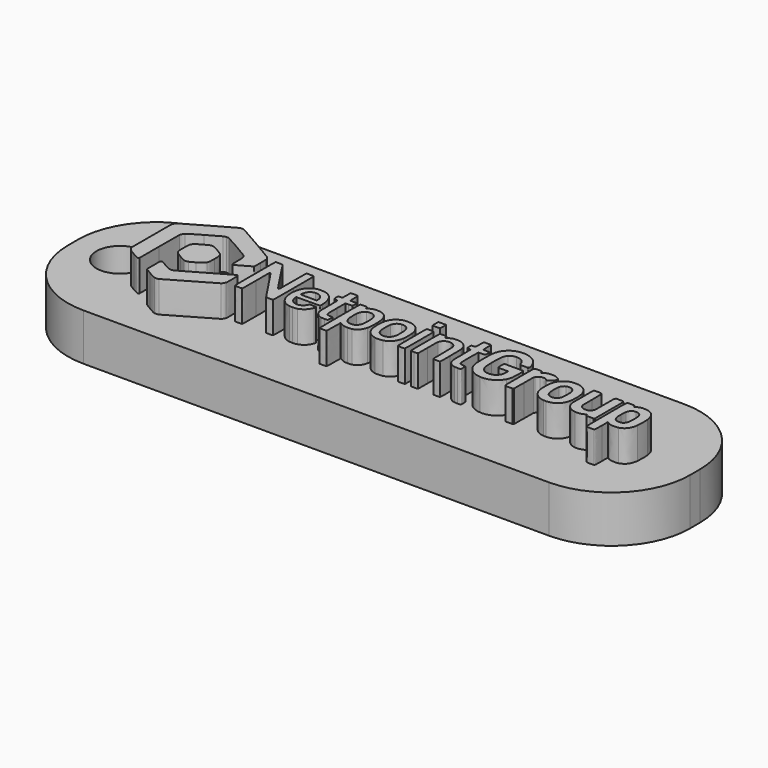
from build123d import *

# Parameters (mm, degrees)
F1_DEPTH = 2
F2_W     = 39.7300348751
F2_H     = 10.813386
F3_DEPTH = 3
F4_R     = 5
F6_D     = 3


# Not quite as in the source:
# - ends of sketch curves that miss each other by under 0.0002 mm in the source are joined
# - a feature names something its author has since deleted; it is built from what else it names


with BuildPart() as f1:
    # F0 (on Top) → F1 (new body)
    with BuildSketch(Plane.XY):
        with BuildLine():
            add(Edge.make_bspline(
                [(-12.934739, -3.423148), (-13.018761, -3.404257), (-12.980204, -3.424206), (-13.418644, -3.171907)],
                knots=[0, 0, 0, 0, 1, 1, 1, 1], degree=3))
            add(Edge.make_bspline(
                [(-12.663873, -3.404841), (-12.743201, -3.434522), (-12.851544, -3.441846), (-12.934739, -3.423148)],
                knots=[0, 0, 0, 0, 1, 1, 1, 1], degree=3))
            add(Edge.make_bspline(
                [(-9.953232, -1.835661), (-10.014995, -1.890099), (-12.572616, -3.370697), (-12.663873, -3.404841)],
                knots=[0, 0, 0, 0, 1, 1, 1, 1], degree=3))
            add(Edge.make_bspline(
                [(-9.811877, -1.614655), (-9.840102, -1.705981), (-9.884035, -1.774669), (-9.953232, -1.835661)],
                knots=[0, 0, 0, 0, 1, 1, 1, 1], degree=3))
            add(Edge.make_bspline(
                [(-9.789869, -1.125945), (-9.789869, -1.509261), (-9.791668, -1.549273), (-9.811877, -1.614655)],
                knots=[0, 0, 0, 0, 1, 1, 1, 1], degree=3))
            add(Edge.make_bspline(
                [(-9.812417, -0.679786), (-9.79074, -0.707343), (-9.789869, -0.724575), (-9.789869, -1.125945)],
                knots=[0, 0, 0, 0, 1, 1, 1, 1], degree=3))
            add(Edge.make_bspline(
                [(-9.869125, -0.643621), (-9.850334, -0.647748), (-9.824817, -0.66402), (-9.812417, -0.679786)],
                knots=[0, 0, 0, 0, 1, 1, 1, 1], degree=3))
            add(Edge.make_bspline(
                [(-11.375308, -1.483263), (-9.765318, -0.553623), (-9.910471, -0.63454), (-9.869125, -0.643621)],
                knots=[0, 0, 0, 0, 1, 1, 1, 1], degree=3))
            add(Edge.make_bspline(
                [(-12.691896, -2.226019), (-12.652934, -2.214563), (-12.167761, -1.940841), (-11.375308, -1.483263)],
                knots=[0, 0, 0, 0, 1, 1, 1, 1], degree=3))
            add(Edge.make_bspline(
                [(-12.983912, -2.221019), (-12.905986, -2.248681), (-12.776437, -2.250898), (-12.691896, -2.226019)],
                knots=[0, 0, 0, 0, 1, 1, 1, 1], degree=3))
            add(Edge.make_bspline(
                [(-13.358996, -2.018025), (-13.186933, -2.117519), (-13.018145, -2.208866), (-12.983912, -2.221019)],
                knots=[0, 0, 0, 0, 1, 1, 1, 1], degree=3))
            add(Edge.make_bspline(
                [(-13.768617, -1.851494), (-13.721476, -1.815301), (-13.68144, -1.831571), (-13.358996, -2.018025)],
                knots=[0, 0, 0, 0, 1, 1, 1, 1], degree=3))
            add(Edge.make_bspline(
                [(-13.812466, -2.408405), (-13.812466, -1.902548), (-13.81101, -1.88404), (-13.768617, -1.851494)],
                knots=[0, 0, 0, 0, 1, 1, 1, 1], degree=3))
            add(Edge.make_bspline(
                [(-13.796813, -2.932975), (-13.809518, -2.908422), (-13.812466, -2.809669), (-13.812466, -2.408405)],
                knots=[0, 0, 0, 0, 1, 1, 1, 1], degree=3))
            add(Edge.make_bspline(
                [(-13.418644, -3.171907), (-13.685045, -3.01856), (-13.785311, -2.955211), (-13.796813, -2.932975)],
                knots=[0, 0, 0, 0, 1, 1, 1, 1], degree=3))
        make_face()
    extrude(amount=F1_DEPTH)



with BuildPart() as f1b:
    # F0 (on Top) → F1, piece 2 (new body)
    with BuildSketch(Plane.XY):
        with BuildLine():
            add(Edge.make_bspline(
                [(-3.094246, -2.529348), (-3.109835, -2.507097), (-3.11169, -2.335221), (-3.11169, -0.912718)],
                knots=[0, 0, 0, 0, 1, 1, 1, 1], degree=3))
            add(Edge.make_bspline(
                [(-2.870782, -2.554235), (-3.070978, -2.554235), (-3.077297, -2.553441), (-3.094246, -2.529348)],
                knots=[0, 0, 0, 0, 1, 1, 1, 1], degree=3))
            add(Edge.make_bspline(
                [(-2.647318, -2.529338), (-2.664267, -2.553547), (-2.670588, -2.554235), (-2.870782, -2.554235)],
                knots=[0, 0, 0, 0, 1, 1, 1, 1], degree=3))
            add(Edge.make_bspline(
                [(-2.629874, -1.993739), (-2.629874, -2.437824), (-2.632149, -2.507682), (-2.647318, -2.529338)],
                knots=[0, 0, 0, 0, 1, 1, 1, 1], degree=3))
            add(Edge.make_bspline(
                [(-2.616427, -1.469597), (-2.626492, -1.479651), (-2.629874, -1.611472), (-2.629874, -1.993739)],
                knots=[0, 0, 0, 0, 1, 1, 1, 1], degree=3))
            add(Edge.make_bspline(
                [(-2.519436, -1.488038), (-2.563105, -1.453941), (-2.59475, -1.447927), (-2.616427, -1.469597)],
                knots=[0, 0, 0, 0, 1, 1, 1, 1], degree=3))
            add(Edge.make_bspline(
                [(-2.293723, -1.603719), (-2.382754, -1.576049), (-2.452487, -1.540309), (-2.519436, -1.488038)],
                knots=[0, 0, 0, 0, 1, 1, 1, 1], degree=3))
            add(Edge.make_bspline(
                [(-2.030406, -1.629622), (-2.187038, -1.629834), (-2.220303, -1.626526), (-2.293723, -1.603719)],
                knots=[0, 0, 0, 0, 1, 1, 1, 1], degree=3))
            add(Edge.make_bspline(
                [(-1.778293, -1.609276), (-1.834176, -1.624727), (-1.892849, -1.629463), (-2.030406, -1.629622)],
                knots=[0, 0, 0, 0, 1, 1, 1, 1], degree=3))
            add(Edge.make_bspline(
                [(-1.247316, -1.022649), (-1.323597, -1.33902), (-1.498066, -1.531777), (-1.778293, -1.609276)],
                knots=[0, 0, 0, 0, 1, 1, 1, 1], degree=3))
            add(Edge.make_bspline(
                [(-1.198527, -0.360448), (-1.192326, -0.683075), (-1.204155, -0.84364), (-1.247316, -1.022649)],
                knots=[0, 0, 0, 0, 1, 1, 1, 1], degree=3))
            add(Edge.make_bspline(
                [(-1.26407, 0.207777), (-1.217128, 0.049678), (-1.204268, -0.061812), (-1.198527, -0.360448)],
                knots=[0, 0, 0, 0, 1, 1, 1, 1], degree=3))
            add(Edge.make_bspline(
                [(-1.621423, 0.665032), (-1.461517, 0.588518), (-1.325404, 0.41435), (-1.26407, 0.207777)],
                knots=[0, 0, 0, 0, 1, 1, 1, 1], degree=3))
            add(Edge.make_bspline(
                [(-1.987661, 0.748273), (-1.821812, 0.742108), (-1.746889, 0.725069), (-1.621423, 0.665032)],
                knots=[0, 0, 0, 0, 1, 1, 1, 1], degree=3))
            add(Edge.make_bspline(
                [(-2.505454, 0.613399), (-2.363918, 0.720529), (-2.223672, 0.75706), (-1.987661, 0.748273)],
                knots=[0, 0, 0, 0, 1, 1, 1, 1], degree=3))
            add(Edge.make_bspline(
                [(-2.607019, 0.568018), (-2.582645, 0.559498), (-2.568071, 0.565901), (-2.505454, 0.613399)],
                knots=[0, 0, 0, 0, 1, 1, 1, 1], degree=3))
            add(Edge.make_bspline(
                [(-2.639002, 0.633698), (-2.635959, 0.585607), (-2.631575, 0.576603), (-2.607019, 0.568018)],
                knots=[0, 0, 0, 0, 1, 1, 1, 1], degree=3))
            add(Edge.make_bspline(
                [(-2.877485, 0.72881), (-2.648098, 0.72881), (-2.644941, 0.727487), (-2.639002, 0.633698)],
                knots=[0, 0, 0, 0, 1, 1, 1, 1], degree=3))
            add(Edge.make_bspline(
                [(-3.094246, 0.703913), (-3.077331, 0.728069), (-3.070753, 0.72881), (-2.877485, 0.72881)],
                knots=[0, 0, 0, 0, 1, 1, 1, 1], degree=3))
            add(Edge.make_bspline(
                [(-3.11169, -0.912718), (-3.11169, 0.509783), (-3.109837, 0.681656), (-3.094246, 0.703913)],
                knots=[0, 0, 0, 0, 1, 1, 1, 1], degree=3))
        make_face()
        with BuildLine():
            add(Edge.make_bspline(
                [(-1.991503, -1.191898), (-1.747455, -1.119423), (-1.652635, -0.872662), (-1.669226, -0.353201)],
                knots=[0, 0, 0, 0, 1, 1, 1, 1], degree=3))
            add(Edge.make_bspline(
                [(-2.323383, -1.186519), (-2.235741, -1.2143), (-2.07574, -1.216875), (-1.991503, -1.191898)],
                knots=[0, 0, 0, 0, 1, 1, 1, 1], degree=3))
            add(Edge.make_bspline(
                [(-2.602575, -0.82304), (-2.560305, -1.010558), (-2.457898, -1.143881), (-2.323383, -1.186519)],
                knots=[0, 0, 0, 0, 1, 1, 1, 1], degree=3))
            add(Edge.make_bspline(
                [(-2.618942, -0.170408), (-2.637084, -0.315021), (-2.62707, -0.714373), (-2.602575, -0.82304)],
                knots=[0, 0, 0, 0, 1, 1, 1, 1], degree=3))
            add(Edge.make_bspline(
                [(-2.357878, 0.291896), (-2.505464, 0.226613), (-2.58732, 0.081658), (-2.618942, -0.170408)],
                knots=[0, 0, 0, 0, 1, 1, 1, 1], degree=3))
            add(Edge.make_bspline(
                [(-1.939523, 0.292425), (-2.052117, 0.34223), (-2.24459, 0.341968), (-2.357878, 0.291896)],
                knots=[0, 0, 0, 0, 1, 1, 1, 1], degree=3))
            add(Edge.make_bspline(
                [(-1.747097, 0.092964), (-1.786426, 0.179112), (-1.863151, 0.258643), (-1.939523, 0.292425)],
                knots=[0, 0, 0, 0, 1, 1, 1, 1], degree=3))
            add(Edge.make_bspline(
                [(-1.669226, -0.353201), (-1.67619, -0.135176), (-1.696766, -0.017286), (-1.747097, 0.092964)],
                knots=[0, 0, 0, 0, 1, 1, 1, 1], degree=3))
        make_face(mode=Mode.SUBTRACT)
    extrude(amount=F1_DEPTH)


with BuildPart() as f1c:
    # F0 (on Top) → F1, piece 3 (new body)
    with BuildSketch(Plane.XY):
        with BuildLine():
            add(Edge.make_bspline(
                [(13.969443, -2.530221), (13.956637, -2.524004), (13.937716, -2.504663), (13.927424, -2.487232)],
                knots=[0, 0, 0, 0, 1, 1, 1, 1], degree=3))
            add(Edge.make_bspline(
                [(14.418843, -2.529645), (14.382354, -2.54626), (14.003518, -2.546737), (13.969443, -2.530221)],
                knots=[0, 0, 0, 0, 1, 1, 1, 1], degree=3))
            add(Edge.make_bspline(
                [(14.48016, -1.966548), (14.48016, -2.495815), (14.479366, -2.502014), (14.418843, -2.529645)],
                knots=[0, 0, 0, 0, 1, 1, 1, 1], degree=3))
            Line((14.48016, -1.966548), (14.48016, -1.478593))
            Line((14.48016, -1.478593), (14.533383, -1.516449))
            add(Edge.make_bspline(
                [(15.012396, -1.649048), (14.793157, -1.649048), (14.673065, -1.615803), (14.533383, -1.516449)],
                knots=[0, 0, 0, 0, 1, 1, 1, 1], degree=3))
            add(Edge.make_bspline(
                [(15.258905, -1.625447), (15.188222, -1.644074), (15.136094, -1.649048), (15.012396, -1.649048)],
                knots=[0, 0, 0, 0, 1, 1, 1, 1], degree=3))
            add(Edge.make_bspline(
                [(15.855107, -0.856687), (15.786633, -1.29838), (15.603337, -1.534729), (15.258905, -1.625447)],
                knots=[0, 0, 0, 0, 1, 1, 1, 1], degree=3))
            add(Edge.make_bspline(
                [(15.860557, -0.049927), (15.882306, -0.204735), (15.878946, -0.703062), (15.855107, -0.856687)],
                knots=[0, 0, 0, 0, 1, 1, 1, 1], degree=3))
            add(Edge.make_bspline(
                [(15.292534, 0.740399), (15.625806, 0.634193), (15.798171, 0.394372), (15.860557, -0.049927)],
                knots=[0, 0, 0, 0, 1, 1, 1, 1], degree=3))
            add(Edge.make_bspline(
                [(14.785685, 0.753311), (14.910825, 0.784955), (15.173715, 0.778261), (15.292534, 0.740399)],
                knots=[0, 0, 0, 0, 1, 1, 1, 1], degree=3))
            add(Edge.make_bspline(
                [(14.520824, 0.632917), (14.591428, 0.686829), (14.677499, 0.725953), (14.785685, 0.753311)],
                knots=[0, 0, 0, 0, 1, 1, 1, 1], degree=3))
            Line((14.520824, 0.632917), (14.468968, 0.593322))
            Line((14.468968, 0.593322), (14.468968, 0.639519))
            add(Edge.make_bspline(
                [(14.436213, 0.718465), (14.461824, 0.692853), (14.468968, 0.675637), (14.468968, 0.639519)],
                knots=[0, 0, 0, 0, 1, 1, 1, 1], degree=3))
            Line((14.436213, 0.718465), (14.40346, 0.75122))
            Line((14.40346, 0.75122), (14.201437, 0.75122))
            add(Edge.make_bspline(
                [(13.971411, 0.738468), (13.989032, 0.746511), (14.074228, 0.75122), (14.201437, 0.75122)],
                knots=[0, 0, 0, 0, 1, 1, 1, 1], degree=3))
            add(Edge.make_bspline(
                [(13.908718, -0.901478), (13.908718, 0.796102), (13.905358, 0.708374), (13.971411, 0.738468)],
                knots=[0, 0, 0, 0, 1, 1, 1, 1], degree=3))
            add(Edge.make_bspline(
                [(13.927424, -2.487232), (13.910173, -2.458046), (13.908718, -2.333144), (13.908718, -0.901478)],
                knots=[0, 0, 0, 0, 1, 1, 1, 1], degree=3))
        make_face()
        with BuildLine():
            add(Edge.make_bspline(
                [(15.075031, -1.101257), (15.176363, -1.055513), (15.239564, -0.966142), (15.283649, -0.806271)],
                knots=[0, 0, 0, 0, 1, 1, 1, 1], degree=3))
            add(Edge.make_bspline(
                [(14.911492, -1.127763), (14.995505, -1.125382), (15.036409, -1.118661), (15.075031, -1.101257)],
                knots=[0, 0, 0, 0, 1, 1, 1, 1], degree=3))
            add(Edge.make_bspline(
                [(14.641961, -1.049901), (14.714782, -1.113999), (14.776184, -1.131737), (14.911492, -1.127763)],
                knots=[0, 0, 0, 0, 1, 1, 1, 1], degree=3))
            add(Edge.make_bspline(
                [(14.511746, -0.822111), (14.541808, -0.93136), (14.57677, -0.992516), (14.641961, -1.049901)],
                knots=[0, 0, 0, 0, 1, 1, 1, 1], degree=3))
            add(Edge.make_bspline(
                [(14.486637, -0.442109), (14.487166, -0.705406), (14.489706, -0.741969), (14.511746, -0.822111)],
                knots=[0, 0, 0, 0, 1, 1, 1, 1], degree=3))
            add(Edge.make_bspline(
                [(14.50566, -0.07342), (14.489177, -0.137981), (14.486028, -0.198967), (14.486637, -0.442109)],
                knots=[0, 0, 0, 0, 1, 1, 1, 1], degree=3))
            add(Edge.make_bspline(
                [(14.874177, 0.255862), (14.667548, 0.245226), (14.563184, 0.151982), (14.50566, -0.07342)],
                knots=[0, 0, 0, 0, 1, 1, 1, 1], degree=3))
            add(Edge.make_bspline(
                [(15.157713, 0.166886), (15.078131, 0.239617), (15.004935, 0.262588), (14.874177, 0.255862)],
                knots=[0, 0, 0, 0, 1, 1, 1, 1], degree=3))
            add(Edge.make_bspline(
                [(15.284178, -0.069083), (15.250261, 0.053554), (15.220065, 0.1099), (15.157713, 0.166886)],
                knots=[0, 0, 0, 0, 1, 1, 1, 1], degree=3))
            add(Edge.make_bspline(
                [(15.283649, -0.806271), (15.312886, -0.700241), (15.313304, -0.174189), (15.284178, -0.069083)],
                knots=[0, 0, 0, 0, 1, 1, 1, 1], degree=3))
        make_face(mode=Mode.SUBTRACT)
    extrude(amount=F1_DEPTH)


with BuildPart() as f1d:
    # F0 (on Top) → F1, piece 4 (new body)
    with BuildSketch(Plane.XY):
        with BuildLine():
            add(Edge.make_bspline(
                [(-15.319538, -2.078617), (-15.580275, -1.928162), (-15.670973, -1.869888), (-15.723821, -1.818868)],
                knots=[0, 0, 0, 0, 1, 1, 1, 1], degree=3))
            add(Edge.make_bspline(
                [(-14.870841, -2.246633), (-14.925169, -2.30096), (-14.95105, -2.291268), (-15.319538, -2.078617)],
                knots=[0, 0, 0, 0, 1, 1, 1, 1], degree=3))
            Line((-14.870841, -2.246633), (-14.843339, -2.21913))
            Line((-14.843339, -2.21913), (-14.843339, -0.657051))
            add(Edge.make_bspline(
                [(-14.832075, 0.965382), (-14.839283, 0.926769), (-14.843339, 0.34231), (-14.843339, -0.657051)],
                knots=[0, 0, 0, 0, 1, 1, 1, 1], degree=3))
            add(Edge.make_bspline(
                [(-14.693636, 1.223883), (-14.759078, 1.160351), (-14.815271, 1.055422), (-14.832075, 0.965382)],
                knots=[0, 0, 0, 0, 1, 1, 1, 1], degree=3))
            add(Edge.make_bspline(
                [(-13.879709, 1.716952), (-14.456598, 1.383514), (-14.64971, 1.266528), (-14.693636, 1.223883)],
                knots=[0, 0, 0, 0, 1, 1, 1, 1], degree=3))
            add(Edge.make_bspline(
                [(-13.04001, 2.194448), (-13.08586, 2.172276), (-13.463724, 1.957392), (-13.879709, 1.716952)],
                knots=[0, 0, 0, 0, 1, 1, 1, 1], degree=3))
            add(Edge.make_bspline(
                [(-12.85963, 2.239422), (-12.942676, 2.235454), (-12.968655, 2.228971), (-13.04001, 2.194448)],
                knots=[0, 0, 0, 0, 1, 1, 1, 1], degree=3))
            add(Edge.make_bspline(
                [(-12.69648, 2.225029), (-12.743918, 2.238681), (-12.790032, 2.242756), (-12.85963, 2.239422)],
                knots=[0, 0, 0, 0, 1, 1, 1, 1], degree=3))
            add(Edge.make_bspline(
                [(-10.982981, 1.24161), (-11.057248, 1.306859), (-12.617411, 2.202275), (-12.69648, 2.225029)],
                knots=[0, 0, 0, 0, 1, 1, 1, 1], degree=3))
            add(Edge.make_bspline(
                [(-10.841973, 1.019116), (-10.868471, 1.104254), (-10.921021, 1.187172), (-10.982981, 1.24161)],
                knots=[0, 0, 0, 0, 1, 1, 1, 1], degree=3))
            add(Edge.make_bspline(
                [(-10.820745, 0.57038), (-10.820745, 0.912378), (-10.822889, 0.957815), (-10.841973, 1.019116)],
                knots=[0, 0, 0, 0, 1, 1, 1, 1], degree=3))
            add(Edge.make_bspline(
                [(-10.804778, 0.158974), (-10.817679, 0.183925), (-10.820745, 0.26295), (-10.820745, 0.57038)],
                knots=[0, 0, 0, 0, 1, 1, 1, 1], degree=3))
            add(Edge.make_bspline(
                [(-10.711785, 0.101324), (-10.745788, 0.101324), (-10.788733, 0.127949), (-10.804778, 0.158974)],
                knots=[0, 0, 0, 0, 1, 1, 1, 1], degree=3))
            add(Edge.make_bspline(
                [(-9.80938, 0.61967), (-9.838929, 0.590121), (-10.689892, 0.101324), (-10.711785, 0.101324)],
                knots=[0, 0, 0, 0, 1, 1, 1, 1], degree=3))
            add(Edge.make_bspline(
                [(-9.792129, 1.119346), (-9.788957, 0.666673), (-9.789907, 0.63914), (-9.80938, 0.61967)],
                knots=[0, 0, 0, 0, 1, 1, 1, 1], degree=3))
            Line((-9.792129, 1.119346), (-9.795487, 1.598416))
            Line((-9.795487, 1.598416), (-9.837583, 1.683562))
            add(Edge.make_bspline(
                [(-9.94403, 1.82731), (-9.898154, 1.785532), (-9.867592, 1.74426), (-9.837583, 1.683562)],
                knots=[0, 0, 0, 0, 1, 1, 1, 1], degree=3))
            add(Edge.make_bspline(
                [(-11.30764, 2.635199), (-10.330074, 2.071433), (-9.992448, 1.871403), (-9.94403, 1.82731)],
                knots=[0, 0, 0, 0, 1, 1, 1, 1], degree=3))
            add(Edge.make_bspline(
                [(-12.669047, 3.408545), (-12.634865, 3.395315), (-12.022232, 3.047306), (-11.30764, 2.635199)],
                knots=[0, 0, 0, 0, 1, 1, 1, 1], degree=3))
            add(Edge.make_bspline(
                [(-12.98331, 3.41119), (-12.89578, 3.441845), (-12.751932, 3.440639), (-12.669047, 3.408545)],
                knots=[0, 0, 0, 0, 1, 1, 1, 1], degree=3))
            add(Edge.make_bspline(
                [(-14.221462, 2.710333), (-13.574373, 3.083933), (-13.017205, 3.399319), (-12.98331, 3.41119)],
                knots=[0, 0, 0, 0, 1, 1, 1, 1], degree=3))
            add(Edge.make_bspline(
                [(-15.532448, 1.954191), (-15.458495, 1.996466), (-14.868551, 2.336731), (-14.221462, 2.710333)],
                knots=[0, 0, 0, 0, 1, 1, 1, 1], degree=3))
            add(Edge.make_bspline(
                [(-15.861696, 1.571439), (-15.827793, 1.73243), (-15.738217, 1.836565), (-15.532448, 1.954191)],
                knots=[0, 0, 0, 0, 1, 1, 1, 1], degree=3))
            add(Edge.make_bspline(
                [(-15.861696, -1.570461), (-15.879346, -1.486551), (-15.879331, 1.48763), (-15.861696, 1.571439)],
                knots=[0, 0, 0, 0, 1, 1, 1, 1], degree=3))
            add(Edge.make_bspline(
                [(-15.723821, -1.818868), (-15.797391, -1.747843), (-15.840859, -1.669527), (-15.861696, -1.570461)],
                knots=[0, 0, 0, 0, 1, 1, 1, 1], degree=3))
        make_face()
    extrude(amount=F1_DEPTH)


with BuildPart() as f1e:
    # F0 (on Top) → F1, piece 5 (new body)
    with BuildSketch(Plane.XY):
        with BuildLine():
            add(Edge.make_bspline(
                [(6.45178, -1.650474), (6.128772, -1.624465), (5.876884, -1.508599), (5.67293, -1.292194)],
                knots=[0, 0, 0, 0, 1, 1, 1, 1], degree=3))
            add(Edge.make_bspline(
                [(7.644658, -1.01608), (7.436155, -1.441268), (6.965051, -1.691815), (6.45178, -1.650474)],
                knots=[0, 0, 0, 0, 1, 1, 1, 1], degree=3))
            add(Edge.make_bspline(
                [(7.768353, -0.19652), (7.768353, -0.670148), (7.747924, -0.80549), (7.644658, -1.01608)],
                knots=[0, 0, 0, 0, 1, 1, 1, 1], degree=3))
            Line((7.768353, -0.19652), (7.768353, 0.139313))
            Line((7.768353, 0.139313), (7.738244, 0.17074))
            Line((7.738244, 0.17074), (7.708135, 0.202165))
            Line((7.708135, 0.202165), (7.13527, 0.202165))
            Line((7.13527, 0.202165), (6.562406, 0.202165))
            Line((6.562406, 0.202165), (6.532297, 0.17074))
            Line((6.532297, 0.17074), (6.502188, 0.139313))
            Line((6.502188, 0.139313), (6.502188, -0.057968))
            Line((6.502188, -0.057968), (6.502188, -0.255247))
            Line((6.502188, -0.255247), (6.536662, -0.284256))
            Line((6.536662, -0.284256), (6.571138, -0.313264))
            Line((6.571138, -0.313264), (6.872812, -0.313264))
            Line((6.872812, -0.313264), (7.174488, -0.313264))
            Line((7.174488, -0.313264), (7.174488, -0.445932))
            add(Edge.make_bspline(
                [(7.000891, -0.936176), (7.125751, -0.80961), (7.174488, -0.671957), (7.174488, -0.445932)],
                knots=[0, 0, 0, 0, 1, 1, 1, 1], degree=3))
            add(Edge.make_bspline(
                [(6.706107, -1.096526), (6.809656, -1.075095), (6.926636, -1.01146), (7.000891, -0.936176)],
                knots=[0, 0, 0, 0, 1, 1, 1, 1], degree=3))
            add(Edge.make_bspline(
                [(6.391589, -1.092531), (6.463321, -1.111634), (6.623334, -1.113645), (6.706107, -1.096526)],
                knots=[0, 0, 0, 0, 1, 1, 1, 1], degree=3))
            add(Edge.make_bspline(
                [(6.061641, -0.852914), (6.118508, -0.957395), (6.254252, -1.055976), (6.391589, -1.092531)],
                knots=[0, 0, 0, 0, 1, 1, 1, 1], degree=3))
            add(Edge.make_bspline(
                [(5.945178, -0.100357), (5.952973, -0.560999), (5.972923, -0.689907), (6.061641, -0.852914)],
                knots=[0, 0, 0, 0, 1, 1, 1, 1], degree=3))
            add(Edge.make_bspline(
                [(6.133157, 0.986215), (5.977622, 0.83068), (5.933716, 0.576897), (5.945178, -0.100357)],
                knots=[0, 0, 0, 0, 1, 1, 1, 1], degree=3))
            add(Edge.make_bspline(
                [(6.518974, 1.150844), (6.357482, 1.141267), (6.236639, 1.089699), (6.133157, 0.986215)],
                knots=[0, 0, 0, 0, 1, 1, 1, 1], degree=3))
            add(Edge.make_bspline(
                [(6.976112, 0.99905), (6.858225, 1.111146), (6.705361, 1.161907), (6.518974, 1.150844)],
                knots=[0, 0, 0, 0, 1, 1, 1, 1], degree=3))
            add(Edge.make_bspline(
                [(7.146938, 0.725503), (7.105698, 0.842473), (7.054418, 0.924589), (6.976112, 0.99905)],
                knots=[0, 0, 0, 0, 1, 1, 1, 1], degree=3))
            add(Edge.make_bspline(
                [(7.201003, 0.621855), (7.187888, 0.631036), (7.164296, 0.676269), (7.146938, 0.725503)],
                knots=[0, 0, 0, 0, 1, 1, 1, 1], degree=3))
            add(Edge.make_bspline(
                [(7.452219, 0.605557), (7.270898, 0.605557), (7.219513, 0.60889), (7.201003, 0.621855)],
                knots=[0, 0, 0, 0, 1, 1, 1, 1], degree=3))
            add(Edge.make_bspline(
                [(7.702787, 0.617675), (7.688708, 0.610134), (7.594076, 0.605557), (7.452219, 0.605557)],
                knots=[0, 0, 0, 0, 1, 1, 1, 1], degree=3))
            add(Edge.make_bspline(
                [(7.741684, 0.668734), (7.732733, 0.647303), (7.715228, 0.624334), (7.702787, 0.617675)],
                knots=[0, 0, 0, 0, 1, 1, 1, 1], degree=3))
            add(Edge.make_bspline(
                [(7.729265, 0.816297), (7.755638, 0.716467), (7.756643, 0.704537), (7.741684, 0.668734)],
                knots=[0, 0, 0, 0, 1, 1, 1, 1], degree=3))
            add(Edge.make_bspline(
                [(7.639998, 1.048165), (7.673313, 0.980376), (7.713482, 0.876035), (7.729265, 0.816297)],
                knots=[0, 0, 0, 0, 1, 1, 1, 1], degree=3))
            add(Edge.make_bspline(
                [(6.781854, 1.676479), (7.17654, 1.607769), (7.470908, 1.39224), (7.639998, 1.048165)],
                knots=[0, 0, 0, 0, 1, 1, 1, 1], degree=3))
            add(Edge.make_bspline(
                [(6.216439, 1.654413), (6.36732, 1.693756), (6.62485, 1.703805), (6.781854, 1.676479)],
                knots=[0, 0, 0, 0, 1, 1, 1, 1], degree=3))
            add(Edge.make_bspline(
                [(5.695195, 1.357267), (5.839101, 1.50247), (6.012221, 1.60116), (6.216439, 1.654413)],
                knots=[0, 0, 0, 0, 1, 1, 1, 1], degree=3))
            add(Edge.make_bspline(
                [(5.368531, 0.627165), (5.409832, 0.951552), (5.505901, 1.166267), (5.695195, 1.357267)],
                knots=[0, 0, 0, 0, 1, 1, 1, 1], degree=3))
            add(Edge.make_bspline(
                [(5.368658, -0.592805), (5.347978, -0.429671), (5.347912, 0.464941), (5.368531, 0.627165)],
                knots=[0, 0, 0, 0, 1, 1, 1, 1], degree=3))
            add(Edge.make_bspline(
                [(5.67293, -1.292194), (5.498333, -1.106943), (5.407308, -0.897716), (5.368658, -0.592805)],
                knots=[0, 0, 0, 0, 1, 1, 1, 1], degree=3))
        make_face()
    extrude(amount=F1_DEPTH)


with BuildPart() as f1f:
    # F0 (on Top) → F1, piece 6 (new body)
    with BuildSketch(Plane.XY):
        with BuildLine():
            add(Edge.make_bspline(
                [(10.485581, -1.646955), (10.08999, -1.601179), (9.797088, -1.361583), (9.680026, -0.988002)],
                knots=[0, 0, 0, 0, 1, 1, 1, 1], degree=3))
            add(Edge.make_bspline(
                [(10.664807, -1.650572), (10.609343, -1.653588), (10.528666, -1.651895), (10.485581, -1.646955)],
                knots=[0, 0, 0, 0, 1, 1, 1, 1], degree=3))
            add(Edge.make_bspline(
                [(11.579453, -0.880843), (11.477195, -1.349378), (11.15058, -1.624243), (10.664807, -1.650572)],
                knots=[0, 0, 0, 0, 1, 1, 1, 1], degree=3))
            add(Edge.make_bspline(
                [(11.579189, 0.009271), (11.627817, -0.213532), (11.627975, -0.658771), (11.579453, -0.880843)],
                knots=[0, 0, 0, 0, 1, 1, 1, 1], degree=3))
            add(Edge.make_bspline(
                [(10.800666, 0.762923), (11.205891, 0.697555), (11.488728, 0.423754), (11.579189, 0.009271)],
                knots=[0, 0, 0, 0, 1, 1, 1, 1], degree=3))
            add(Edge.make_bspline(
                [(10.340606, 0.74636), (10.43041, 0.771151), (10.69144, 0.780549), (10.800666, 0.762923)],
                knots=[0, 0, 0, 0, 1, 1, 1, 1], degree=3))
            add(Edge.make_bspline(
                [(9.914126, 0.498842), (10.046106, 0.631174), (10.157482, 0.695811), (10.340606, 0.74636)],
                knots=[0, 0, 0, 0, 1, 1, 1, 1], degree=3))
            add(Edge.make_bspline(
                [(9.699658, 0.169108), (9.753545, 0.312568), (9.800789, 0.385204), (9.914126, 0.498842)],
                knots=[0, 0, 0, 0, 1, 1, 1, 1], degree=3))
            add(Edge.make_bspline(
                [(9.620314, -0.374886), (9.626373, -0.095512), (9.642936, 0.018118), (9.699658, 0.169108)],
                knots=[0, 0, 0, 0, 1, 1, 1, 1], degree=3))
            add(Edge.make_bspline(
                [(9.680026, -0.988002), (9.631371, -0.832726), (9.614208, -0.656506), (9.620314, -0.374886)],
                knots=[0, 0, 0, 0, 1, 1, 1, 1], degree=3))
        make_face()
        with BuildLine():
            add(Edge.make_bspline(
                [(10.795377, -1.095479), (10.914791, -1.040382), (10.983472, -0.945603), (11.025241, -0.778264)],
                knots=[0, 0, 0, 0, 1, 1, 1, 1], degree=3))
            add(Edge.make_bspline(
                [(10.460438, -1.108107), (10.546869, -1.14226), (10.707069, -1.136219), (10.795377, -1.095479)],
                knots=[0, 0, 0, 0, 1, 1, 1, 1], degree=3))
            add(Edge.make_bspline(
                [(10.206044, -0.759), (10.2384, -0.931948), (10.32889, -1.05613), (10.460438, -1.108107)],
                knots=[0, 0, 0, 0, 1, 1, 1, 1], degree=3))
            add(Edge.make_bspline(
                [(10.212473, -0.069377), (10.175101, -0.223362), (10.171807, -0.576059), (10.206044, -0.759)],
                knots=[0, 0, 0, 0, 1, 1, 1, 1], degree=3))
            add(Edge.make_bspline(
                [(10.43348, 0.222924), (10.321849, 0.17059), (10.246538, 0.070982), (10.212473, -0.069377)],
                knots=[0, 0, 0, 0, 1, 1, 1, 1], degree=3))
            add(Edge.make_bspline(
                [(10.614418, 0.252595), (10.510571, 0.252595), (10.489338, 0.249102), (10.43348, 0.222924)],
                knots=[0, 0, 0, 0, 1, 1, 1, 1], degree=3))
            add(Edge.make_bspline(
                [(10.79421, 0.223451), (10.739642, 0.249036), (10.717737, 0.252595), (10.614418, 0.252595)],
                knots=[0, 0, 0, 0, 1, 1, 1, 1], degree=3))
            add(Edge.make_bspline(
                [(11.025506, -0.094761), (10.983874, 0.074485), (10.917693, 0.165531), (10.79421, 0.223451)],
                knots=[0, 0, 0, 0, 1, 1, 1, 1], degree=3))
            add(Edge.make_bspline(
                [(11.025241, -0.778264), (11.05347, -0.665179), (11.053658, -0.209127), (11.025506, -0.094761)],
                knots=[0, 0, 0, 0, 1, 1, 1, 1], degree=3))
        make_face(mode=Mode.SUBTRACT)
    extrude(amount=F1_DEPTH)


with BuildPart() as f1g:
    # F0 (on Top) → F1, piece 7 (new body)
    with BuildSketch(Plane.XY):
        with BuildLine():
            add(Edge.make_bspline(
                [(12.508083, -1.646839), (12.301544, -1.620883), (12.153962, -1.551528), (12.020141, -1.417567)],
                knots=[0, 0, 0, 0, 1, 1, 1, 1], degree=3))
            add(Edge.make_bspline(
                [(13.131309, -1.501611), (12.962782, -1.614324), (12.712783, -1.67258), (12.508083, -1.646839)],
                knots=[0, 0, 0, 0, 1, 1, 1, 1], degree=3))
            Line((13.131309, -1.501611), (13.166263, -1.478222))
            Line((13.166263, -1.478222), (13.173592, -1.52399))
            add(Edge.make_bspline(
                [(13.210305, -1.596999), (13.192129, -1.580171), (13.178116, -1.552279), (13.173592, -1.52399)],
                knots=[0, 0, 0, 0, 1, 1, 1, 1], degree=3))
            add(Edge.make_bspline(
                [(13.451817, -1.62424), (13.24269, -1.62424), (13.239283, -1.623976), (13.210305, -1.596999)],
                knots=[0, 0, 0, 0, 1, 1, 1, 1], degree=3))
            Line((13.451817, -1.62424), (13.663939, -1.62424))
            Line((13.663939, -1.62424), (13.696692, -1.591488))
            Line((13.696692, -1.591488), (13.729444, -1.558732))
            Line((13.729444, -1.558732), (13.729444, -0.43651))
            Line((13.729444, -0.43651), (13.729444, 0.685715))
            Line((13.729444, 0.685715), (13.696692, 0.718468))
            Line((13.696692, 0.718468), (13.663939, 0.75122))
            Line((13.663939, 0.75122), (13.450359, 0.75122))
            Line((13.450359, 0.75122), (13.23678, 0.75122))
            Line((13.23678, 0.75122), (13.200185, 0.718534))
            Line((13.200185, 0.718534), (13.163593, 0.685845))
            Line((13.163593, 0.685845), (13.157984, -0.074221))
            add(Edge.make_bspline(
                [(13.126798, -0.897562), (13.152356, -0.834351), (13.152383, -0.833515), (13.157984, -0.074221)],
                knots=[0, 0, 0, 0, 1, 1, 1, 1], degree=3))
            add(Edge.make_bspline(
                [(12.947487, -1.094182), (13.025589, -1.055833), (13.092444, -0.982525), (13.126798, -0.897562)],
                knots=[0, 0, 0, 0, 1, 1, 1, 1], degree=3))
            add(Edge.make_bspline(
                [(12.749002, -1.125617), (12.873647, -1.125617), (12.888136, -1.123236), (12.947487, -1.094182)],
                knots=[0, 0, 0, 0, 1, 1, 1, 1], degree=3))
            add(Edge.make_bspline(
                [(12.558068, -1.095807), (12.610133, -1.123292), (12.625037, -1.125617), (12.749002, -1.125617)],
                knots=[0, 0, 0, 0, 1, 1, 1, 1], degree=3))
            add(Edge.make_bspline(
                [(12.383551, -0.900608), (12.416193, -0.981615), (12.48273, -1.05604), (12.558068, -1.095807)],
                knots=[0, 0, 0, 0, 1, 1, 1, 1], degree=3))
            Line((12.383551, -0.900608), (12.356826, -0.834287))
            Line((12.356826, -0.834287), (12.351217, -0.077949))
            add(Edge.make_bspline(
                [(12.335844, 0.698412), (12.341215, 0.687406), (12.348121, 0.338037), (12.351217, -0.077949)],
                knots=[0, 0, 0, 0, 1, 1, 1, 1], degree=3))
            add(Edge.make_bspline(
                [(12.066565, 0.75122), (12.272074, 0.75122), (12.314119, 0.742965), (12.335844, 0.698412)],
                knots=[0, 0, 0, 0, 1, 1, 1, 1], degree=3))
            add(Edge.make_bspline(
                [(11.841068, 0.737833), (11.860277, 0.74659), (11.938379, 0.75122), (12.066565, 0.75122)],
                knots=[0, 0, 0, 0, 1, 1, 1, 1], degree=3))
            add(Edge.make_bspline(
                [(11.779754, -0.080492), (11.779754, 0.726101), (11.778431, 0.709324), (11.841068, 0.737833)],
                knots=[0, 0, 0, 0, 1, 1, 1, 1], degree=3))
            add(Edge.make_bspline(
                [(11.79121, -0.918621), (11.78449, -0.862823), (11.779754, -0.517232), (11.779754, -0.080492)],
                knots=[0, 0, 0, 0, 1, 1, 1, 1], degree=3))
            add(Edge.make_bspline(
                [(12.020141, -1.417567), (11.885285, -1.282573), (11.817216, -1.134216), (11.79121, -0.918621)],
                knots=[0, 0, 0, 0, 1, 1, 1, 1], degree=3))
        make_face()
    extrude(amount=F1_DEPTH)


with BuildPart() as f1h:
    # F0 (on Top) → F1, piece 8 (new body)
    with BuildSketch(Plane.XY):
        with BuildLine():
            add(Edge.make_bspline(
                [(-5.757964, -1.624693), (-6.110688, -1.560359), (-6.367827, -1.327918), (-6.488657, -0.964179)],
                knots=[0, 0, 0, 0, 1, 1, 1, 1], degree=3))
            add(Edge.make_bspline(
                [(-5.537572, -1.630421), (-5.630014, -1.632538), (-5.72919, -1.629892), (-5.757964, -1.624693)],
                knots=[0, 0, 0, 0, 1, 1, 1, 1], degree=3))
            add(Edge.make_bspline(
                [(-5.269069, -1.596769), (-5.354104, -1.622063), (-5.39526, -1.627212), (-5.537572, -1.630421)],
                knots=[0, 0, 0, 0, 1, 1, 1, 1], degree=3))
            add(Edge.make_bspline(
                [(-4.664116, -1.01609), (-4.776995, -1.316183), (-4.979657, -1.510713), (-5.269069, -1.596769)],
                knots=[0, 0, 0, 0, 1, 1, 1, 1], degree=3))
            add(Edge.make_bspline(
                [(-4.654114, -0.871562), (-4.628804, -0.899528), (-4.630728, -0.927325), (-4.664116, -1.01609)],
                knots=[0, 0, 0, 0, 1, 1, 1, 1], degree=3))
            add(Edge.make_bspline(
                [(-4.859265, -0.851083), (-4.692713, -0.851083), (-4.670665, -0.8532), (-4.654114, -0.871562)],
                knots=[0, 0, 0, 0, 1, 1, 1, 1], degree=3))
            add(Edge.make_bspline(
                [(-5.064777, -0.865079), (-5.051431, -0.855184), (-4.990998, -0.851083), (-4.859265, -0.851083)],
                knots=[0, 0, 0, 0, 1, 1, 1, 1], degree=3))
            add(Edge.make_bspline(
                [(-5.122995, -0.961343), (-5.101371, -0.916102), (-5.075174, -0.872784), (-5.064777, -0.865079)],
                knots=[0, 0, 0, 0, 1, 1, 1, 1], degree=3))
            add(Edge.make_bspline(
                [(-5.650065, -1.235541), (-5.423813, -1.268135), (-5.218599, -1.161378), (-5.122995, -0.961343)],
                knots=[0, 0, 0, 0, 1, 1, 1, 1], degree=3))
            add(Edge.make_bspline(
                [(-6.088318, -0.748393), (-6.063831, -1.011854), (-5.894246, -1.200362), (-5.650065, -1.235541)],
                knots=[0, 0, 0, 0, 1, 1, 1, 1], degree=3))
            add(Edge.make_bspline(
                [(-6.081228, -0.655244), (-6.091261, -0.667335), (-6.093327, -0.694495), (-6.088318, -0.748393)],
                knots=[0, 0, 0, 0, 1, 1, 1, 1], degree=3))
            add(Edge.make_bspline(
                [(-5.348209, -0.638178), (-5.978332, -0.638178), (-6.068814, -0.640295), (-6.081228, -0.655244)],
                knots=[0, 0, 0, 0, 1, 1, 1, 1], degree=3))
            add(Edge.make_bspline(
                [(-4.602782, -0.619578), (-4.626872, -0.636458), (-4.696414, -0.638178), (-5.348209, -0.638178)],
                knots=[0, 0, 0, 0, 1, 1, 1, 1], degree=3))
            add(Edge.make_bspline(
                [(-4.583157, -0.431896), (-4.576223, -0.600673), (-4.576257, -0.601001), (-4.602782, -0.619578)],
                knots=[0, 0, 0, 0, 1, 1, 1, 1], degree=3))
            add(Edge.make_bspline(
                [(-4.719302, 0.197201), (-4.635019, 0.023032), (-4.594075, -0.166156), (-4.583157, -0.431896)],
                knots=[0, 0, 0, 0, 1, 1, 1, 1], degree=3))
            add(Edge.make_bspline(
                [(-5.270988, 0.6643), (-5.01683, 0.590634), (-4.835329, 0.436959), (-4.719302, 0.197201)],
                knots=[0, 0, 0, 0, 1, 1, 1, 1], degree=3))
            add(Edge.make_bspline(
                [(-5.571186, 0.689223), (-5.382736, 0.689488), (-5.348267, 0.686577), (-5.270988, 0.6643)],
                knots=[0, 0, 0, 0, 1, 1, 1, 1], degree=3))
            add(Edge.make_bspline(
                [(-5.890529, 0.653079), (-5.785906, 0.688242), (-5.780433, 0.688861), (-5.571186, 0.689223)],
                knots=[0, 0, 0, 0, 1, 1, 1, 1], degree=3))
            add(Edge.make_bspline(
                [(-6.222393, 0.456289), (-6.119318, 0.552293), (-6.026308, 0.607448), (-5.890529, 0.653079)],
                knots=[0, 0, 0, 0, 1, 1, 1, 1], degree=3))
            add(Edge.make_bspline(
                [(-6.562697, -0.470125), (-6.562697, -0.066607), (-6.447707, 0.246432), (-6.222393, 0.456289)],
                knots=[0, 0, 0, 0, 1, 1, 1, 1], degree=3))
            add(Edge.make_bspline(
                [(-6.488657, -0.964179), (-6.540774, -0.807292), (-6.562697, -0.661004), (-6.562697, -0.470125)],
                knots=[0, 0, 0, 0, 1, 1, 1, 1], degree=3))
        make_face()
        with BuildLine():
            add(Edge.make_bspline(
                [(-5.068306, -0.276839), (-5.055706, -0.256969), (-5.054497, -0.23622), (-5.062591, -0.178795)],
                knots=[0, 0, 0, 0, 1, 1, 1, 1], degree=3))
            Line((-5.068306, -0.276839), (-5.084286, -0.302051))
            Line((-5.084286, -0.302051), (-5.575676, -0.302051))
            add(Edge.make_bspline(
                [(-6.081228, -0.284986), (-6.068938, -0.299802), (-6.002084, -0.302051), (-5.575676, -0.302051)],
                knots=[0, 0, 0, 0, 1, 1, 1, 1], degree=3))
            add(Edge.make_bspline(
                [(-6.053826, -0.03768), (-6.087183, -0.129577), (-6.101673, -0.26035), (-6.081228, -0.284986)],
                knots=[0, 0, 0, 0, 1, 1, 1, 1], degree=3))
            add(Edge.make_bspline(
                [(-5.610405, 0.300074), (-5.823586, 0.287295), (-5.97877, 0.169097), (-6.053826, -0.03768)],
                knots=[0, 0, 0, 0, 1, 1, 1, 1], degree=3))
            add(Edge.make_bspline(
                [(-5.136789, 0.04782), (-5.226643, 0.220995), (-5.398912, 0.312748), (-5.610405, 0.300074)],
                knots=[0, 0, 0, 0, 1, 1, 1, 1], degree=3))
            add(Edge.make_bspline(
                [(-5.062591, -0.178795), (-5.075876, -0.084527), (-5.089139, -0.044014), (-5.136789, 0.04782)],
                knots=[0, 0, 0, 0, 1, 1, 1, 1], degree=3))
        make_face(mode=Mode.SUBTRACT)
    extrude(amount=F1_DEPTH)


with BuildPart() as f1i:
    # F0 (on Top) → F1, piece 9 (new body)
    with BuildSketch(Plane.XY):
        with BuildLine():
            add(Edge.make_bspline(
                [(-0.269431, -1.624365), (-0.702642, -1.546389), (-0.969939, -1.250154), (-1.039889, -0.770496)],
                knots=[0, 0, 0, 0, 1, 1, 1, 1], degree=3))
            add(Edge.make_bspline(
                [(0.198019, -1.603241), (0.09942, -1.629619), (-0.172055, -1.641904), (-0.269431, -1.624365)],
                knots=[0, 0, 0, 0, 1, 1, 1, 1], degree=3))
            add(Edge.make_bspline(
                [(0.872359, -0.797841), (0.807503, -1.222505), (0.572683, -1.502961), (0.198019, -1.603241)],
                knots=[0, 0, 0, 0, 1, 1, 1, 1], degree=3))
            add(Edge.make_bspline(
                [(0.878373, -0.121068), (0.897674, -0.269), (0.894248, -0.654521), (0.872359, -0.797841)],
                knots=[0, 0, 0, 0, 1, 1, 1, 1], degree=3))
            add(Edge.make_bspline(
                [(0.18749, 0.724029), (0.587957, 0.612957), (0.819567, 0.329647), (0.878373, -0.121068)],
                knots=[0, 0, 0, 0, 1, 1, 1, 1], degree=3))
            add(Edge.make_bspline(
                [(-0.300431, 0.734877), (-0.18303, 0.758637), (0.084192, 0.752684), (0.18749, 0.724029)],
                knots=[0, 0, 0, 0, 1, 1, 1, 1], degree=3))
            add(Edge.make_bspline(
                [(-0.755124, 0.50175), (-0.632006, 0.618188), (-0.472183, 0.700132), (-0.300431, 0.734877)],
                knots=[0, 0, 0, 0, 1, 1, 1, 1], degree=3))
            add(Edge.make_bspline(
                [(-1.039644, -0.111565), (-1.003243, 0.154299), (-0.910016, 0.355258), (-0.755124, 0.50175)],
                knots=[0, 0, 0, 0, 1, 1, 1, 1], degree=3))
            add(Edge.make_bspline(
                [(-1.039889, -0.770496), (-1.058047, -0.645983), (-1.057894, -0.244909), (-1.039644, -0.111565)],
                knots=[0, 0, 0, 0, 1, 1, 1, 1], degree=3))
        make_face()
        with BuildLine():
            add(Edge.make_bspline(
                [(0.129431, -1.167014), (0.26878, -1.098413), (0.350066, -0.987068), (0.392427, -0.80676)],
                knots=[0, 0, 0, 0, 1, 1, 1, 1], degree=3))
            add(Edge.make_bspline(
                [(-0.063471, -1.206993), (0.044064, -1.204135), (0.0613, -1.200563), (0.129431, -1.167014)],
                knots=[0, 0, 0, 0, 1, 1, 1, 1], degree=3))
            add(Edge.make_bspline(
                [(-0.360629, -1.126258), (-0.26256, -1.1938), (-0.200603, -1.210633), (-0.063471, -1.206993)],
                knots=[0, 0, 0, 0, 1, 1, 1, 1], degree=3))
            add(Edge.make_bspline(
                [(-0.553377, -0.811877), (-0.513699, -0.968936), (-0.458624, -1.058765), (-0.360629, -1.126258)],
                knots=[0, 0, 0, 0, 1, 1, 1, 1], degree=3))
            add(Edge.make_bspline(
                [(-0.553487, -0.064413), (-0.582817, -0.189394), (-0.582759, -0.695672), (-0.553377, -0.811877)],
                knots=[0, 0, 0, 0, 1, 1, 1, 1], degree=3))
            add(Edge.make_bspline(
                [(-0.158841, 0.324678), (-0.366089, 0.295298), (-0.500072, 0.163202), (-0.553487, -0.064413)],
                knots=[0, 0, 0, 0, 1, 1, 1, 1], degree=3))
            add(Edge.make_bspline(
                [(0.336937, 0.087151), (0.252244, 0.261135), (0.056036, 0.355139), (-0.158841, 0.324678)],
                knots=[0, 0, 0, 0, 1, 1, 1, 1], degree=3))
            add(Edge.make_bspline(
                [(0.412284, -0.442111), (0.412284, -0.128808), (0.399976, -0.04235), (0.336937, 0.087151)],
                knots=[0, 0, 0, 0, 1, 1, 1, 1], degree=3))
            add(Edge.make_bspline(
                [(0.392427, -0.80676), (0.408651, -0.737706), (0.412284, -0.670971), (0.412284, -0.442111)],
                knots=[0, 0, 0, 0, 1, 1, 1, 1], degree=3))
        make_face(mode=Mode.SUBTRACT)
    extrude(amount=F1_DEPTH)


with BuildPart() as f1j:
    # F0 (on Top) → F1, piece 10 (new body)
    with BuildSketch(Plane.XY):
        with BuildLine():
            add(Edge.make_bspline(
                [(8.259999, 0.75122), (8.387208, 0.75122), (8.472393, 0.746511), (8.490025, 0.738468)],
                knots=[0, 0, 0, 0, 1, 1, 1, 1], degree=3))
            Line((8.259999, 0.75122), (8.057974, 0.75122))
            Line((8.057974, 0.75122), (8.025221, 0.718468))
            Line((8.025221, 0.718468), (7.992468, 0.685715))
            Line((7.992468, 0.685715), (7.992468, -0.43651))
            Line((7.992468, -0.43651), (7.992468, -1.558732))
            Line((7.992468, -1.558732), (8.025221, -1.591488))
            Line((8.025221, -1.591488), (8.057964, -1.62436))
            Line((8.057964, -1.62436), (8.271543, -1.62436))
            Line((8.271543, -1.62436), (8.485122, -1.62436))
            Line((8.485122, -1.62436), (8.521717, -1.591673))
            Line((8.521717, -1.591673), (8.558309, -1.558984))
            Line((8.558309, -1.558984), (8.563918, -0.804522))
            Line((8.563918, -0.804522), (8.569527, -0.050057))
            Line((8.569527, -0.050057), (8.60469, 0.024159))
            add(Edge.make_bspline(
                [(8.786226, 0.221329), (8.70756, 0.1827), (8.650384, 0.120597), (8.60469, 0.024159)],
                knots=[0, 0, 0, 0, 1, 1, 1, 1], degree=3))
            add(Edge.make_bspline(
                [(8.9617, 0.252478), (8.861855, 0.252478), (8.842744, 0.249092), (8.786226, 0.221329)],
                knots=[0, 0, 0, 0, 1, 1, 1, 1], degree=3))
            add(Edge.make_bspline(
                [(9.206951, 0.169555), (9.11705, 0.241231), (9.083787, 0.252478), (8.9617, 0.252478)],
                knots=[0, 0, 0, 0, 1, 1, 1, 1], degree=3))
            add(Edge.make_bspline(
                [(9.295721, 0.134826), (9.262002, 0.134826), (9.239436, 0.143663), (9.206951, 0.169555)],
                knots=[0, 0, 0, 0, 1, 1, 1, 1], degree=3))
            add(Edge.make_bspline(
                [(9.501382, 0.293904), (9.348233, 0.142062), (9.338877, 0.134826), (9.295721, 0.134826)],
                knots=[0, 0, 0, 0, 1, 1, 1, 1], degree=3))
            add(Edge.make_bspline(
                [(9.659904, 0.553778), (9.691146, 0.494149), (9.672472, 0.463542), (9.501382, 0.293904)],
                knots=[0, 0, 0, 0, 1, 1, 1, 1], degree=3))
            add(Edge.make_bspline(
                [(9.304315, 0.757499), (9.441385, 0.728442), (9.622865, 0.624469), (9.659904, 0.553778)],
                knots=[0, 0, 0, 0, 1, 1, 1, 1], degree=3))
            add(Edge.make_bspline(
                [(8.896682, 0.755647), (8.996755, 0.777978), (9.203606, 0.778983), (9.304315, 0.757499)],
                knots=[0, 0, 0, 0, 1, 1, 1, 1], degree=3))
            add(Edge.make_bspline(
                [(8.589884, 0.621564), (8.648119, 0.66598), (8.808038, 0.735872), (8.896682, 0.755647)],
                knots=[0, 0, 0, 0, 1, 1, 1, 1], degree=3))
            Line((8.589884, 0.621564), (8.552718, 0.593217))
            Line((8.552718, 0.593217), (8.552718, 0.622905))
            add(Edge.make_bspline(
                [(8.490025, 0.738468), (8.52182, 0.723995), (8.552718, 0.667027), (8.552718, 0.622905)],
                knots=[0, 0, 0, 0, 1, 1, 1, 1], degree=3))
        make_face()
    extrude(amount=F1_DEPTH)


with BuildPart() as f1k:
    # F0 (on Top) → F1, piece 11 (new body)
    with BuildSketch(Plane.XY):
        with BuildLine():
            add(Edge.make_bspline(
                [(-9.255895, -1.592546), (-9.272969, -1.573681), (-9.27444, -1.444909), (-9.27444, 0.031379)],
                knots=[0, 0, 0, 0, 1, 1, 1, 1], degree=3))
            add(Edge.make_bspline(
                [(-9.026191, -1.613006), (-9.216528, -1.613006), (-9.239178, -1.61089), (-9.255895, -1.592546)],
                knots=[0, 0, 0, 0, 1, 1, 1, 1], degree=3))
            add(Edge.make_bspline(
                [(-8.792623, -1.590596), (-8.813448, -1.611419), (-8.829972, -1.613006), (-9.026191, -1.613006)],
                knots=[0, 0, 0, 0, 1, 1, 1, 1], degree=3))
            add(Edge.make_bspline(
                [(-8.770213, -0.50895), (-8.770213, -1.553245), (-8.770504, -1.568501), (-8.792623, -1.590596)],
                knots=[0, 0, 0, 0, 1, 1, 1, 1], degree=3))
            Line((-8.770213, -0.50895), (-8.770213, 0.550283))
            Line((-8.770213, 0.550283), (-8.745001, 0.560072))
            add(Edge.make_bspline(
                [(-8.698419, 0.556236), (-8.712339, 0.565099), (-8.728579, 0.566449), (-8.745001, 0.560072)],
                knots=[0, 0, 0, 0, 1, 1, 1, 1], degree=3))
            add(Edge.make_bspline(
                [(-7.978402, -0.521179), (-8.362658, 0.06391), (-8.686665, 0.548748), (-8.698419, 0.556236)],
                knots=[0, 0, 0, 0, 1, 1, 1, 1], degree=3))
            add(Edge.make_bspline(
                [(-7.260902, -1.598983), (-7.271274, -1.591284), (-7.594147, -1.106268), (-7.978402, -0.521179)],
                knots=[0, 0, 0, 0, 1, 1, 1, 1], degree=3))
            add(Edge.make_bspline(
                [(-6.825484, -1.597131), (-6.854905, -1.618642), (-7.232285, -1.620282), (-7.260902, -1.598983)],
                knots=[0, 0, 0, 0, 1, 1, 1, 1], degree=3))
            add(Edge.make_bspline(
                [(-6.800819, 0.018182), (-6.80368, -1.550374), (-6.804153, -1.581534), (-6.825484, -1.597131)],
                knots=[0, 0, 0, 0, 1, 1, 1, 1], degree=3))
            add(Edge.make_bspline(
                [(-6.815086, 1.643811), (-6.799817, 1.620501), (-6.798229, 1.439656), (-6.800819, 0.018182)],
                knots=[0, 0, 0, 0, 1, 1, 1, 1], degree=3))
            add(Edge.make_bspline(
                [(-7.053867, 1.670031), (-6.833898, 1.670031), (-6.832139, 1.669819), (-6.815086, 1.643811)],
                knots=[0, 0, 0, 0, 1, 1, 1, 1], degree=3))
            add(Edge.make_bspline(
                [(-7.288913, 1.65659), (-7.279361, 1.666142), (-7.211282, 1.670031), (-7.053867, 1.670031)],
                knots=[0, 0, 0, 0, 1, 1, 1, 1], degree=3))
            add(Edge.make_bspline(
                [(-7.302359, 0.58825), (-7.302359, 1.393782), (-7.299179, 1.646324), (-7.288913, 1.65659)],
                knots=[0, 0, 0, 0, 1, 1, 1, 1], degree=3))
            add(Edge.make_bspline(
                [(-7.323936, -0.486172), (-7.302928, -0.467149), (-7.302359, -0.43883), (-7.302359, 0.58825)],
                knots=[0, 0, 0, 0, 1, 1, 1, 1], degree=3))
            add(Edge.make_bspline(
                [(-7.365954, -0.501915), (-7.354712, -0.504032), (-7.335803, -0.496914), (-7.323936, -0.486172)],
                knots=[0, 0, 0, 0, 1, 1, 1, 1], degree=3))
            add(Edge.make_bspline(
                [(-8.185369, 0.712009), (-7.381919, -0.509585), (-7.390116, -0.497444), (-7.365954, -0.501915)],
                knots=[0, 0, 0, 0, 1, 1, 1, 1], degree=3))
            Line((-8.185369, 0.712009), (-8.811785, 1.664432))
            Line((-8.811785, 1.664432), (-9.025266, 1.667475))
            add(Edge.make_bspline(
                [(-9.256594, 1.652658), (-9.24129, 1.667951), (-9.208328, 1.670068), (-9.025266, 1.667475)],
                knots=[0, 0, 0, 0, 1, 1, 1, 1], degree=3))
            add(Edge.make_bspline(
                [(-9.27444, 0.031379), (-9.27444, 1.48319), (-9.272746, 1.6365), (-9.256594, 1.652658)],
                knots=[0, 0, 0, 0, 1, 1, 1, 1], degree=3))
        make_face()
    extrude(amount=F1_DEPTH)


with BuildPart() as f1l:
    # F0 (on Top) → F1, piece 12 (new body)
    with BuildSketch(Plane.XY):
        with BuildLine():
            add(Edge.make_bspline(
                [(-3.749523, -1.595959), (-3.932789, -1.562791), (-4.083157, -1.449653), (-4.166163, -1.282478)],
                knots=[0, 0, 0, 0, 1, 1, 1, 1], degree=3))
            add(Edge.make_bspline(
                [(-3.512264, -1.612025), (-3.597002, -1.611496), (-3.703768, -1.604246), (-3.749523, -1.595959)],
                knots=[0, 0, 0, 0, 1, 1, 1, 1], degree=3))
            add(Edge.make_bspline(
                [(-3.313375, -1.407885), (-3.313375, -1.62142), (-3.305543, -1.613382), (-3.512264, -1.612025)],
                knots=[0, 0, 0, 0, 1, 1, 1, 1], degree=3))
            add(Edge.make_bspline(
                [(-3.327382, -1.229704), (-3.317661, -1.242087), (-3.313375, -1.29661), (-3.313375, -1.407885)],
                knots=[0, 0, 0, 0, 1, 1, 1, 1], degree=3))
            add(Edge.make_bspline(
                [(-3.465269, -1.207215), (-3.369251, -1.210813), (-3.338239, -1.215893), (-3.327382, -1.229704)],
                knots=[0, 0, 0, 0, 1, 1, 1, 1], degree=3))
            add(Edge.make_bspline(
                [(-3.749599, -1.047195), (-3.716596, -1.161302), (-3.647139, -1.200391), (-3.465269, -1.207215)],
                knots=[0, 0, 0, 0, 1, 1, 1, 1], degree=3))
            add(Edge.make_bspline(
                [(-3.759267, -0.324472), (-3.761648, -0.813279), (-3.758949, -1.014876), (-3.749599, -1.047195)],
                knots=[0, 0, 0, 0, 1, 1, 1, 1], degree=3))
            Line((-3.759267, -0.324472), (-3.755973, 0.35343))
            Line((-3.755973, 0.35343), (-3.550555, 0.359039))
            add(Edge.make_bspline(
                [(-3.329256, 0.386392), (-3.343695, 0.366627), (-3.363798, 0.36414), (-3.550555, 0.359039)],
                knots=[0, 0, 0, 0, 1, 1, 1, 1], degree=3))
            add(Edge.make_bspline(
                [(-3.313376, 0.547983), (-3.313376, 0.445005), (-3.317562, 0.40241), (-3.329256, 0.386392)],
                knots=[0, 0, 0, 0, 1, 1, 1, 1], degree=3))
            add(Edge.make_bspline(
                [(-3.542574, 0.728805), (-3.300078, 0.728805), (-3.313376, 0.739282), (-3.313376, 0.547983)],
                knots=[0, 0, 0, 0, 1, 1, 1, 1], degree=3))
            add(Edge.make_bspline(
                [(-3.74813, 0.742246), (-3.738719, 0.732827), (-3.677053, 0.728805), (-3.542574, 0.728805)],
                knots=[0, 0, 0, 0, 1, 1, 1, 1], degree=3))
            add(Edge.make_bspline(
                [(-3.761576, 1.04789), (-3.761576, 0.835564), (-3.757901, 0.752017), (-3.74813, 0.742246)],
                knots=[0, 0, 0, 0, 1, 1, 1, 1], degree=3))
            add(Edge.make_bspline(
                [(-3.77902, 1.36499), (-3.764317, 1.344009), (-3.761576, 1.294217), (-3.761576, 1.04789)],
                knots=[0, 0, 0, 0, 1, 1, 1, 1], degree=3))
            add(Edge.make_bspline(
                [(-4.008328, 1.389888), (-3.802094, 1.389888), (-3.795999, 1.389358), (-3.77902, 1.36499)],
                knots=[0, 0, 0, 0, 1, 1, 1, 1], degree=3))
            add(Edge.make_bspline(
                [(-4.231793, 1.368218), (-4.220953, 1.388459), (-4.206327, 1.389888), (-4.008328, 1.389888)],
                knots=[0, 0, 0, 0, 1, 1, 1, 1], degree=3))
            add(Edge.make_bspline(
                [(-4.243392, 1.051115), (-4.243392, 1.233334), (-4.238947, 1.354849), (-4.231793, 1.368218)],
                knots=[0, 0, 0, 0, 1, 1, 1, 1], degree=3))
            add(Edge.make_bspline(
                [(-4.256838, 0.742243), (-4.247062, 0.752006), (-4.243392, 0.836279), (-4.243392, 1.051115)],
                knots=[0, 0, 0, 0, 1, 1, 1, 1], degree=3))
            add(Edge.make_bspline(
                [(-4.373856, 0.728802), (-4.30824, 0.728802), (-4.265356, 0.733724), (-4.256838, 0.742243)],
                knots=[0, 0, 0, 0, 1, 1, 1, 1], degree=3))
            add(Edge.make_bspline(
                [(-4.512312, 0.543567), (-4.512312, 0.726733), (-4.510778, 0.728802), (-4.373856, 0.728802)],
                knots=[0, 0, 0, 0, 1, 1, 1, 1], degree=3))
            add(Edge.make_bspline(
                [(-4.375961, 0.360717), (-4.512508, 0.36585), (-4.512312, 0.365585), (-4.512312, 0.543567)],
                knots=[0, 0, 0, 0, 1, 1, 1, 1], degree=3))
            add(Edge.make_bspline(
                [(-4.257399, 0.345344), (-4.265103, 0.351641), (-4.318455, 0.358573), (-4.375961, 0.360717)],
                knots=[0, 0, 0, 0, 1, 1, 1, 1], degree=3))
            add(Edge.make_bspline(
                [(-4.243003, -0.339842), (-4.243294, 0.185176), (-4.246485, 0.336417), (-4.257399, 0.345344)],
                knots=[0, 0, 0, 0, 1, 1, 1, 1], degree=3))
            add(Edge.make_bspline(
                [(-4.166163, -1.282478), (-4.240189, -1.133393), (-4.242559, -1.104316), (-4.243003, -0.339842)],
                knots=[0, 0, 0, 0, 1, 1, 1, 1], degree=3))
        make_face()
    extrude(amount=F1_DEPTH)


with BuildPart() as f1m:
    # F0 (on Top) → F1, piece 13 (new body)
    with BuildSketch(Plane.XY):
        with BuildLine():
            add(Edge.make_bspline(
                [(1.16236, -1.597018), (1.141114, -1.581486), (1.140542, -1.554949), (1.13765, -0.448662)],
                knots=[0, 0, 0, 0, 1, 1, 1, 1], degree=3))
            add(Edge.make_bspline(
                [(1.378056, -1.612914), (1.228252, -1.612914), (1.179161, -1.609289), (1.16236, -1.597018)],
                knots=[0, 0, 0, 0, 1, 1, 1, 1], degree=3))
            add(Edge.make_bspline(
                [(1.594412, -1.590503), (1.57373, -1.611194), (1.557063, -1.612914), (1.378056, -1.612914)],
                knots=[0, 0, 0, 0, 1, 1, 1, 1], degree=3))
            add(Edge.make_bspline(
                [(1.616823, -0.444482), (1.616823, -1.553152), (1.616532, -1.56839), (1.594412, -1.590503)],
                knots=[0, 0, 0, 0, 1, 1, 1, 1], degree=3))
            add(Edge.make_bspline(
                [(1.599379, 0.704029), (1.614883, 0.681884), (1.616823, 0.554336), (1.616823, -0.444482)],
                knots=[0, 0, 0, 0, 1, 1, 1, 1], degree=3))
            add(Edge.make_bspline(
                [(1.380881, 0.728927), (1.575944, 0.728927), (1.582456, 0.728133), (1.599379, 0.704029)],
                knots=[0, 0, 0, 0, 1, 1, 1, 1], degree=3))
            add(Edge.make_bspline(
                [(1.157259, 0.706358), (1.178203, 0.727286), (1.194298, 0.728927), (1.380881, 0.728927)],
                knots=[0, 0, 0, 0, 1, 1, 1, 1], degree=3))
            add(Edge.make_bspline(
                [(1.13765, -0.448662), (1.134719, 0.673481), (1.134899, 0.683995), (1.157259, 0.706358)],
                knots=[0, 0, 0, 0, 1, 1, 1, 1], degree=3))
        make_face()
    extrude(amount=F1_DEPTH)


with BuildPart() as f1n:
    # F0 (on Top) → F1, piece 14 (new body)
    with BuildSketch(Plane.XY):
        with BuildLine():
            add(Edge.make_bspline(
                [(1.994991, -1.600828), (1.976518, -1.590059), (1.975383, -1.522939), (1.975383, -0.441844)],
                knots=[0, 0, 0, 0, 1, 1, 1, 1], degree=3))
            add(Edge.make_bspline(
                [(2.207888, -1.612604), (2.097556, -1.61239), (2.006186, -1.607365), (1.994991, -1.600828)],
                knots=[0, 0, 0, 0, 1, 1, 1, 1], degree=3))
            add(Edge.make_bspline(
                [(2.423584, -1.590538), (2.402878, -1.611255), (2.386486, -1.612922), (2.207888, -1.612604)],
                knots=[0, 0, 0, 0, 1, 1, 1, 1], degree=3))
            add(Edge.make_bspline(
                [(2.446158, -0.831401), (2.445989, -1.553076), (2.445523, -1.568588), (2.423584, -1.590538)],
                knots=[0, 0, 0, 0, 1, 1, 1, 1], degree=3))
            add(Edge.make_bspline(
                [(2.463264, -0.022808), (2.449058, -0.083072), (2.446299, -0.213572), (2.446158, -0.831401)],
                knots=[0, 0, 0, 0, 1, 1, 1, 1], degree=3))
            add(Edge.make_bspline(
                [(3.000311, 0.324765), (2.737891, 0.361963), (2.52085, 0.221495), (2.463264, -0.022808)],
                knots=[0, 0, 0, 0, 1, 1, 1, 1], degree=3))
            add(Edge.make_bspline(
                [(3.372681, -0.007644), (3.31515, 0.189097), (3.193919, 0.297317), (3.000311, 0.324765)],
                knots=[0, 0, 0, 0, 1, 1, 1, 1], degree=3))
            add(Edge.make_bspline(
                [(3.395271, -0.828599), (3.392001, -0.159306), (3.389402, -0.064823), (3.372681, -0.007644)],
                knots=[0, 0, 0, 0, 1, 1, 1, 1], degree=3))
            add(Edge.make_bspline(
                [(3.417641, -1.598941), (3.400599, -1.586162), (3.398642, -1.518812), (3.395271, -0.828599)],
                knots=[0, 0, 0, 0, 1, 1, 1, 1], degree=3))
            add(Edge.make_bspline(
                [(3.630263, -1.612937), (3.492537, -1.612937), (3.430904, -1.608889), (3.417641, -1.598941)],
                knots=[0, 0, 0, 0, 1, 1, 1, 1], degree=3))
            add(Edge.make_bspline(
                [(3.846619, -1.590527), (3.825937, -1.611218), (3.809269, -1.612937), (3.630263, -1.612937)],
                knots=[0, 0, 0, 0, 1, 1, 1, 1], degree=3))
            add(Edge.make_bspline(
                [(3.868937, -0.80898), (3.869064, -1.553242), (3.868593, -1.568556), (3.846619, -1.590527)],
                knots=[0, 0, 0, 0, 1, 1, 1, 1], degree=3))
            add(Edge.make_bspline(
                [(3.857647, 0.047897), (3.864026, -0.007782), (3.868884, -0.37651), (3.868937, -0.80898)],
                knots=[0, 0, 0, 0, 1, 1, 1, 1], degree=3))
            add(Edge.make_bspline(
                [(3.336792, 0.713832), (3.635349, 0.616675), (3.819445, 0.381299), (3.857647, 0.047897)],
                knots=[0, 0, 0, 0, 1, 1, 1, 1], degree=3))
            add(Edge.make_bspline(
                [(2.846833, 0.730395), (2.985777, 0.763587), (3.206866, 0.756113), (3.336792, 0.713832)],
                knots=[0, 0, 0, 0, 1, 1, 1, 1], degree=3))
            add(Edge.make_bspline(
                [(2.544201, 0.593822), (2.623033, 0.650927), (2.745478, 0.706186), (2.846833, 0.730395)],
                knots=[0, 0, 0, 0, 1, 1, 1, 1], degree=3))
            add(Edge.make_bspline(
                [(2.487214, 0.560829), (2.493508, 0.560829), (2.519151, 0.575672), (2.544201, 0.593822)],
                knots=[0, 0, 0, 0, 1, 1, 1, 1], degree=3))
            add(Edge.make_bspline(
                [(2.434789, 0.642921), (2.434789, 0.599413), (2.459429, 0.560829), (2.487214, 0.560829)],
                knots=[0, 0, 0, 0, 1, 1, 1, 1], degree=3))
            add(Edge.make_bspline(
                [(2.208216, 0.728905), (2.424219, 0.728905), (2.434789, 0.724884), (2.434789, 0.642921)],
                knots=[0, 0, 0, 0, 1, 1, 1, 1], degree=3))
            add(Edge.make_bspline(
                [(1.997058, 0.717317), (2.009546, 0.724011), (2.099027, 0.728905), (2.208216, 0.728905)],
                knots=[0, 0, 0, 0, 1, 1, 1, 1], degree=3))
            add(Edge.make_bspline(
                [(1.975383, -0.441844), (1.975383, 0.681249), (1.975833, 0.705963), (1.997058, 0.717317)],
                knots=[0, 0, 0, 0, 1, 1, 1, 1], degree=3))
        make_face()
    extrude(amount=F1_DEPTH)


with BuildPart() as f1o:
    # F0 (on Top) → F1, piece 15 (new body)
    with BuildSketch(Plane.XY):
        with BuildLine():
            add(Edge.make_bspline(
                [(4.768198, -1.600563), (4.521172, -1.559402), (4.348657, -1.400781), (4.275972, -1.147983)],
                knots=[0, 0, 0, 0, 1, 1, 1, 1], degree=3))
            add(Edge.make_bspline(
                [(4.983049, -1.611675), (4.897256, -1.610882), (4.800576, -1.60596), (4.768198, -1.600563)],
                knots=[0, 0, 0, 0, 1, 1, 1, 1], degree=3))
            add(Edge.make_bspline(
                [(5.180018, -1.411698), (5.180018, -1.624195), (5.190633, -1.613419), (4.983049, -1.611675)],
                knots=[0, 0, 0, 0, 1, 1, 1, 1], degree=3))
            add(Edge.make_bspline(
                [(5.166011, -1.229776), (5.175774, -1.242132), (5.180018, -1.297268), (5.180018, -1.411698)],
                knots=[0, 0, 0, 0, 1, 1, 1, 1], degree=3))
            add(Edge.make_bspline(
                [(5.02875, -1.206625), (5.123068, -1.210779), (5.155294, -1.216203), (5.166011, -1.229776)],
                knots=[0, 0, 0, 0, 1, 1, 1, 1], degree=3))
            add(Edge.make_bspline(
                [(4.866102, -1.184664), (4.888873, -1.194216), (4.957501, -1.203503), (5.02875, -1.206625)],
                knots=[0, 0, 0, 0, 1, 1, 1, 1], degree=3))
            add(Edge.make_bspline(
                [(4.743696, -1.044634), (4.758656, -1.098505), (4.815332, -1.163342), (4.866102, -1.184664)],
                knots=[0, 0, 0, 0, 1, 1, 1, 1], degree=3))
            add(Edge.make_bspline(
                [(4.745257, 0.345651), (4.727453, 0.327845), (4.725977, -0.980856), (4.743696, -1.044634)],
                knots=[0, 0, 0, 0, 1, 1, 1, 1], degree=3))
            add(Edge.make_bspline(
                [(4.944454, 0.359092), (4.814921, 0.359092), (4.754634, 0.355017), (4.745257, 0.345651)],
                knots=[0, 0, 0, 0, 1, 1, 1, 1], degree=3))
            add(Edge.make_bspline(
                [(5.180011, 0.540927), (5.180011, 0.349456), (5.192494, 0.359092), (4.944454, 0.359092)],
                knots=[0, 0, 0, 0, 1, 1, 1, 1], degree=3))
            add(Edge.make_bspline(
                [(4.950813, 0.728858), (5.194153, 0.728858), (5.180011, 0.740447), (5.180011, 0.540927)],
                knots=[0, 0, 0, 0, 1, 1, 1, 1], degree=3))
            add(Edge.make_bspline(
                [(4.745257, 0.742299), (4.754668, 0.73288), (4.816334, 0.728858), (4.950813, 0.728858)],
                knots=[0, 0, 0, 0, 1, 1, 1, 1], degree=3))
            add(Edge.make_bspline(
                [(4.731811, 1.051173), (4.731811, 0.836337), (4.735478, 0.752075), (4.745257, 0.742299)],
                knots=[0, 0, 0, 0, 1, 1, 1, 1], degree=3))
            add(Edge.make_bspline(
                [(4.720212, 1.368274), (4.727366, 1.354912), (4.731811, 1.233392), (4.731811, 1.051173)],
                knots=[0, 0, 0, 0, 1, 1, 1, 1], degree=3))
            add(Edge.make_bspline(
                [(4.498913, 1.389784), (4.694865, 1.389954), (4.709373, 1.388461), (4.720212, 1.368274)],
                knots=[0, 0, 0, 0, 1, 1, 1, 1], degree=3))
            add(Edge.make_bspline(
                [(4.272406, 1.378989), (4.281651, 1.384837), (4.383579, 1.389679), (4.498913, 1.389784)],
                knots=[0, 0, 0, 0, 1, 1, 1, 1], degree=3))
            add(Edge.make_bspline(
                [(4.252271, 1.063132), (4.255071, 1.319762), (4.258277, 1.370068), (4.272406, 1.378989)],
                knots=[0, 0, 0, 0, 1, 1, 1, 1], degree=3))
            add(Edge.make_bspline(
                [(4.236894, 0.74337), (4.244651, 0.75271), (4.250128, 0.866661), (4.252271, 1.063132)],
                knots=[0, 0, 0, 0, 1, 1, 1, 1], degree=3))
            add(Edge.make_bspline(
                [(4.130236, 0.728845), (4.194037, 0.728845), (4.228767, 0.733581), (4.236894, 0.74337)],
                knots=[0, 0, 0, 0, 1, 1, 1, 1], degree=3))
            add(Edge.make_bspline(
                [(3.992282, 0.549806), (3.992282, 0.734673), (3.987792, 0.728845), (4.130236, 0.728845)],
                knots=[0, 0, 0, 0, 1, 1, 1, 1], degree=3))
            add(Edge.make_bspline(
                [(4.133466, 0.359079), (3.992533, 0.359079), (3.992282, 0.359343), (3.992282, 0.549806)],
                knots=[0, 0, 0, 0, 1, 1, 1, 1], degree=3))
            add(Edge.make_bspline(
                [(4.236798, 0.344685), (4.228847, 0.354263), (4.194244, 0.359079), (4.133466, 0.359079)],
                knots=[0, 0, 0, 0, 1, 1, 1, 1], degree=3))
            add(Edge.make_bspline(
                [(4.252696, -0.375235), (4.250024, 0.102539), (4.244894, 0.334933), (4.236798, 0.344685)],
                knots=[0, 0, 0, 0, 1, 1, 1, 1], degree=3))
            add(Edge.make_bspline(
                [(4.275972, -1.147983), (4.258792, -1.088237), (4.256202, -1.002208), (4.252696, -0.375235)],
                knots=[0, 0, 0, 0, 1, 1, 1, 1], degree=3))
        make_face()
    extrude(amount=F1_DEPTH)


with BuildPart() as f1p:
    # F0 (on Top) → F1, piece 16 (new body)
    with BuildSketch(Plane.XY):
        with BuildLine():
            add(Edge.make_bspline(
                [(-12.947102, -1.036088), (-13.02237, -1.014894), (-13.028845, -1.011561), (-13.335252, -0.835819)],
                knots=[0, 0, 0, 0, 1, 1, 1, 1], degree=3))
            add(Edge.make_bspline(
                [(-12.675159, -1.024525), (-12.754025, -1.051169), (-12.875224, -1.056328), (-12.947102, -1.036088)],
                knots=[0, 0, 0, 0, 1, 1, 1, 1], degree=3))
            add(Edge.make_bspline(
                [(-12.344611, -0.847471), (-12.495598, -0.934443), (-12.644345, -1.014114), (-12.675159, -1.024525)],
                knots=[0, 0, 0, 0, 1, 1, 1, 1], degree=3))
            add(Edge.make_bspline(
                [(-11.907415, -0.498952), (-11.962125, -0.61081), (-12.036047, -0.669738), (-12.344611, -0.847471)],
                knots=[0, 0, 0, 0, 1, 1, 1, 1], degree=3))
            add(Edge.make_bspline(
                [(-11.851757, 0.004849), (-11.851587, -0.34035), (-11.857916, -0.397743), (-11.907415, -0.498952)],
                knots=[0, 0, 0, 0, 1, 1, 1, 1], degree=3))
            add(Edge.make_bspline(
                [(-12.305394, 0.825156), (-11.87009, 0.573333), (-11.852038, 0.540689), (-11.851757, 0.004849)],
                knots=[0, 0, 0, 0, 1, 1, 1, 1], degree=3))
            add(Edge.make_bspline(
                [(-12.613775, 0.998614), (-12.579746, 0.981654), (-12.440974, 0.903589), (-12.305394, 0.825156)],
                knots=[0, 0, 0, 0, 1, 1, 1, 1], degree=3))
            add(Edge.make_bspline(
                [(-12.987454, 1.024569), (-12.869499, 1.065553), (-12.728344, 1.055753), (-12.613775, 0.998614)],
                knots=[0, 0, 0, 0, 1, 1, 1, 1], degree=3))
            add(Edge.make_bspline(
                [(-13.313787, 0.849066), (-13.159749, 0.936752), (-13.0129, 1.015727), (-12.987454, 1.024569)],
                knots=[0, 0, 0, 0, 1, 1, 1, 1], degree=3))
            add(Edge.make_bspline(
                [(-13.759561, 0.485724), (-13.698769, 0.614071), (-13.634311, 0.666609), (-13.313787, 0.849066)],
                knots=[0, 0, 0, 0, 1, 1, 1, 1], degree=3))
            Line((-13.759561, 0.485724), (-13.795659, 0.409514))
            Line((-13.795659, 0.409514), (-13.80126, 0.067759))
            add(Edge.make_bspline(
                [(-13.750932, -0.499862), (-13.803511, -0.393145), (-13.807988, -0.342649), (-13.80126, 0.067759)],
                knots=[0, 0, 0, 0, 1, 1, 1, 1], degree=3))
            add(Edge.make_bspline(
                [(-13.335252, -0.835819), (-13.632612, -0.665263), (-13.693808, -0.615805), (-13.750932, -0.499862)],
                knots=[0, 0, 0, 0, 1, 1, 1, 1], degree=3))
        make_face()
    extrude(amount=F1_DEPTH)


with BuildPart() as f1q:
    # F0 (on Top) → F1, piece 17 (new body)
    with BuildSketch(Plane.XY):
        with BuildLine():
            add(Edge.make_bspline(
                [(1.135402, 1.209934), (1.128604, 1.222634), (1.123802, 1.317416), (1.123802, 1.438835)],
                knots=[0, 0, 0, 0, 1, 1, 1, 1], degree=3))
            add(Edge.make_bspline(
                [(1.375915, 1.188257), (1.161062, 1.188257), (1.146289, 1.189579), (1.135402, 1.209934)],
                knots=[0, 0, 0, 0, 1, 1, 1, 1], degree=3))
            add(Edge.make_bspline(
                [(1.616428, 1.209926), (1.60554, 1.189579), (1.590766, 1.188257), (1.375915, 1.188257)],
                knots=[0, 0, 0, 0, 1, 1, 1, 1], degree=3))
            add(Edge.make_bspline(
                [(1.628027, 1.434764), (1.628027, 1.316146), (1.623201, 1.222581), (1.616428, 1.209926)],
                knots=[0, 0, 0, 0, 1, 1, 1, 1], degree=3))
            add(Edge.make_bspline(
                [(1.616428, 1.659599), (1.623201, 1.646951), (1.628027, 1.553379), (1.628027, 1.434764)],
                knots=[0, 0, 0, 0, 1, 1, 1, 1], degree=3))
            add(Edge.make_bspline(
                [(1.381923, 1.681268), (1.590836, 1.681268), (1.605557, 1.679945), (1.616428, 1.659599)],
                knots=[0, 0, 0, 0, 1, 1, 1, 1], degree=3))
            add(Edge.make_bspline(
                [(1.14141, 1.663673), (1.156237, 1.67849), (1.194223, 1.681268), (1.381923, 1.681268)],
                knots=[0, 0, 0, 0, 1, 1, 1, 1], degree=3))
            add(Edge.make_bspline(
                [(1.123802, 1.438835), (1.123802, 1.612286), (1.126673, 1.648936), (1.14141, 1.663673)],
                knots=[0, 0, 0, 0, 1, 1, 1, 1], degree=3))
        make_face()
    extrude(amount=F1_DEPTH)


with BuildPart() as f1_1:
    add(f1.part)

    add(f1b.part)  # F3 merges F1b

    add(f1c.part)  # F3 merges F1c

    add(f1d.part)  # F3 merges F1d

    add(f1e.part)  # F3 merges F1e

    add(f1f.part)  # F3 merges F1f

    add(f1g.part)  # F3 merges F1g

    add(f1h.part)  # F3 merges F1h

    add(f1i.part)  # F3 merges F1i

    add(f1j.part)  # F3 merges F1j

    add(f1k.part)  # F3 merges F1k

    add(f1l.part)  # F3 merges F1l

    add(f1m.part)  # F3 merges F1m

    add(f1n.part)  # F3 merges F1n

    add(f1o.part)  # F3 merges F1o

    add(f1p.part)  # F3 merges F1p

    add(f1q.part)  # F3 merges F1q
    # F2 (on face) → F3 (join)
    with BuildSketch(Plane(origin=(0, 0, 0), x_dir=(1, 0, 0), z_dir=(0, 0, -1))):
        with Locations((-1.0099104375, -0.001852)):
            Rectangle(F2_W, F2_H)
    extrude(amount=F3_DEPTH)

    # F4
    f4_edges = [f1_1.edges().sort_by_distance(p)[0] for p in [
        (-20.874928, 5.408545, -1.5),
        (-20.874928, -5.404841, -1.5),
        (18.855107, -5.404841, -1.5),
        (18.855107, 5.408545, -1.5),
    ]]
    fillet(f4_edges, radius=F4_R)

    # F6 (through all)
    with Locations(Plane.XY):
        with Locations((-17.8749278751, 0.001852)):
            Hole(F6_D / 2)


solid = f1_1.part
